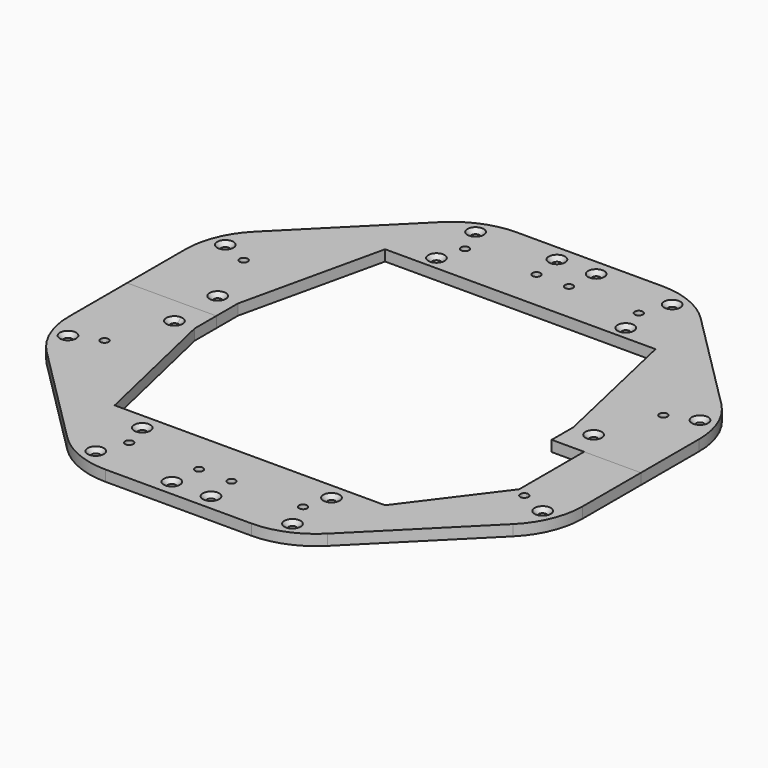
from build123d import *

# Parameters (mm, degrees)
F0_R      = 1.5
F1_DEPTH  = 4
F2_DEPTH  = 4
F3_R      = 30
F3_2_R    = 30
F4_R      = 1.5
F5_DEPTH  = 25
F6_R      = 1.5
F7_DEPTH  = 25
F8_SIZE   = 1.5
F8_2_SIZE = 1.5


with BuildPart() as f1:
    # F0 (on Top) → F1 (new body)
    with BuildSketch(Plane.XY):
        Polygon((0, 0), (95, 0), (95, 39.3502884254), (39.3502884254, 95), (-39.3502884254, 95), (-95, 39.3502884254), (-95, 0), align=None)
        with Locations((-77.6058807309, 32.1454083187)):
            Circle(F0_R, mode=Mode.SUBTRACT)
        with Locations((-87.7685555886, 36.3549260747)):
            Circle(F0_R, mode=Mode.SUBTRACT)
        with Locations((-32.1454083187, 77.6058807309)):
            Circle(F0_R, mode=Mode.SUBTRACT)
        with Locations((-36.3549260747, 87.7685555886)):
            Circle(F0_R, mode=Mode.SUBTRACT)
        with Locations((-6, 78)):
            Circle(F0_R, mode=Mode.SUBTRACT)
        with Locations((-7.25, 89)):
            Circle(F0_R, mode=Mode.SUBTRACT)
        with Locations((77.6058807309, 32.1454083187)):
            Circle(F0_R, mode=Mode.SUBTRACT)
        with Locations((87.7685555886, 36.3549260747)):
            Circle(F0_R, mode=Mode.SUBTRACT)
        with Locations((6, 78)):
            Circle(F0_R, mode=Mode.SUBTRACT)
        with Locations((7.25, 89)):
            Circle(F0_R, mode=Mode.SUBTRACT)
        with Locations((32.1454083187, 77.6058807309)):
            Circle(F0_R, mode=Mode.SUBTRACT)
        with Locations((36.3549260747, 87.7685555886)):
            Circle(F0_R, mode=Mode.SUBTRACT)
    extrude(amount=F1_DEPTH)

    # F3
    f3_edges = [f1.edges().sort_by_distance(p)[0] for p in [
        (95, 39.350288, 2),
        (39.350288, 95, 2),
        (-39.350288, 95, 2),
        (-95, 39.350288, 2),
    ]]
    fillet(f3_edges, radius=F3_R)


with BuildPart() as f2:
    # F0 (on Top) → F2 (new body)
    with BuildSketch(Plane.XY):
        Polygon((-39.3502884254, -95), (39.3502884254, -95), (95, -39.3502884254), (95, 0), (0, 0), (-95, 0), (-95, -39.3502884254), align=None)
        with Locations((-36.3549260747, -87.7685555886)):
            Circle(F0_R, mode=Mode.SUBTRACT)
        with Locations((-32.1454083187, -77.6058807309)):
            Circle(F0_R, mode=Mode.SUBTRACT)
        with Locations((-7.25, -89)):
            Circle(F0_R, mode=Mode.SUBTRACT)
        with Locations((-6, -78)):
            Circle(F0_R, mode=Mode.SUBTRACT)
        with Locations((-87.7685555886, -36.3549260747)):
            Circle(F0_R, mode=Mode.SUBTRACT)
        with Locations((-77.6058807309, -32.1454083187)):
            Circle(F0_R, mode=Mode.SUBTRACT)
        with Locations((7.25, -89)):
            Circle(F0_R, mode=Mode.SUBTRACT)
        with Locations((6, -78)):
            Circle(F0_R, mode=Mode.SUBTRACT)
        with Locations((36.3549260747, -87.7685555886)):
            Circle(F0_R, mode=Mode.SUBTRACT)
        with Locations((32.1454083187, -77.6058807309)):
            Circle(F0_R, mode=Mode.SUBTRACT)
        with Locations((87.7685555886, -36.3549260747)):
            Circle(F0_R, mode=Mode.SUBTRACT)
        with Locations((77.6058807309, -32.1454083187)):
            Circle(F0_R, mode=Mode.SUBTRACT)
    extrude(amount=F2_DEPTH)

    # F3#2
    f3_2_edges = [f2.edges().sort_by_distance(p)[0] for p in [
        (-95, -39.350288, 2),
        (95, -39.350288, 2),
        (-39.350288, -95, 2),
        (39.350288, -95, 2),
    ]]
    fillet(f3_2_edges, radius=F3_2_R)


with BuildPart() as f5_tool:
    # F4 (on face) → F5 (new body)
    with BuildSketch(Plane.XY.offset(4)):
        with Locations((-35, 68)):
            Circle(F4_R)
        with Locations((35, 68)):
            Circle(F4_R)
        with Locations((35, -68)):
            Circle(F4_R)
        with Locations((-35, -68)):
            Circle(F4_R)
    extrude(amount=-F5_DEPTH)


with BuildPart() as f1_1:
    add(f1.part)

    # F5: cut by f5_tool
    add(f5_tool.part, mode=Mode.SUBTRACT)


with BuildPart() as f2_1:
    add(f2.part)

    # F5: cut by f5_tool
    add(f5_tool.part, mode=Mode.SUBTRACT)


with BuildPart() as f7_tool:
    # F6 (on face) → F7 (new body)
    with BuildSketch(Plane.XY.offset(4)):
        with BuildLine():
            ThreePointArc((-68, 10), (-70.5606601718, 11.0606601718), (-69.5, 8.5))
            ThreePointArc((-69.5, 8.5), (-68.4393398282, 8.9393398282), (-68, 10))
        make_face()
        Polygon((0, 63), (-50, 63), (-50, 0), (0, 0), (50, 0), (50, 63), align=None)
        Polygon((-50, 0), (-50, 63), (-62, 10), (-62, 0), align=None)
        Polygon((0, 0), (-50, 0), (-50, -62), (50, -62), (50, 0), align=None)
        Polygon((-50, -62), (-50, 0), (-62, 0), (-62, -10), align=None)
        Polygon((62, 10), (50, 63), (50, 0), (62, 0), align=None)
        with BuildLine():
            ThreePointArc((-68, -10), (-68.4393398282, -8.9393398282), (-69.5, -8.5))
            ThreePointArc((-69.5, -8.5), (-70.5606601718, -11.0606601718), (-68, -10))
        make_face()
        Polygon((62, 0), (50, 0), (50, -62), (74, -30), (74, 0), align=None)
        with Locations((69.5, -10)):
            Circle(F6_R, mode=Mode.SUBTRACT)
        with Locations((69.5, 10)):
            Circle(F6_R)
        with Locations((69.5, -10)):
            Circle(F6_R)
    extrude(amount=-F7_DEPTH)


with BuildPart() as f1_2:
    add(f1_1.part)

    # F7: cut by f7_tool
    add(f7_tool.part, mode=Mode.SUBTRACT)

    # F8
    f8_edges = [f1_2.edges().sort_by_distance(p)[0] for p in [
        (-36.5, 68, 4),
        (33.5, 68, 4),
        (-89.268556, 36.354926, 4),
        (-37.854926, 87.768556, 4),
        (-8.75, 89, 4),
        (5.75, 89, 4),
        (34.854926, 87.768556, 4),
        (86.268556, 36.354926, 4),
        (-79.105881, 32.145408, 0),
        (76.105881, 32.145408, 0),
        (30.645408, 77.605881, 0),
        (4.5, 78, 0),
        (-7.5, 78, 0),
        (-33.645408, 77.605881, 0),
        (-69.5, 11.5, 4),
        (68, 10, 4),
    ]]
    chamfer(f8_edges, length=F8_SIZE)


with BuildPart() as f2_2:
    add(f2_1.part)

    # F7: cut by f7_tool
    add(f7_tool.part, mode=Mode.SUBTRACT)

    # F8#2
    f8_2_edges = [f2_2.edges().sort_by_distance(p)[0] for p in [
        (-36.5, -68, 4),
        (33.5, -68, 4),
        (34.854926, -87.768556, 4),
        (5.75, -89, 4),
        (-8.75, -89, 4),
        (-37.854926, -87.768556, 4),
        (-89.268556, -36.354926, 4),
        (86.268556, -36.354926, 4),
        (-79.105881, -32.145408, 0),
        (-33.645408, -77.605881, 0),
        (-7.5, -78, 0),
        (4.5, -78, 0),
        (30.645408, -77.605881, 0),
        (76.105881, -32.145408, 0),
        (-71, -10, 4),
    ]]
    chamfer(f8_2_edges, length=F8_2_SIZE)


solid = Compound([f1_2.part, f2_2.part])
